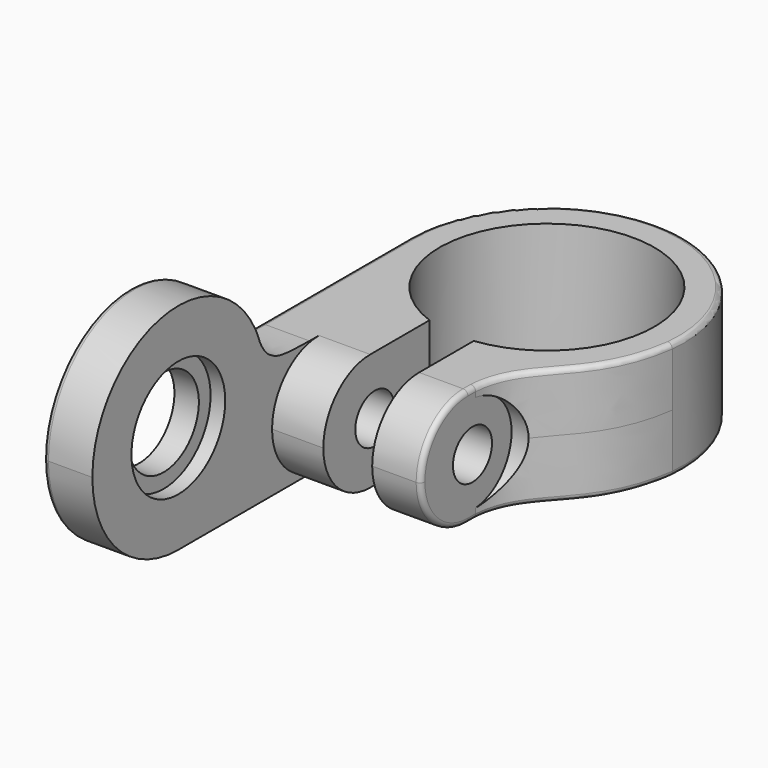
from build123d import *

# Parameters (mm, degrees)
F1_DEPTH     = 6
F3_DEPTH     = 5
F4_R         = 2.5
F5_DEPTH     = 28.0010001
F4_R_2       = 5
F6_DEPTH     = 6
F7_R         = 5
F8_DEPTH     = 7.7510001
F9_R         = 4.5
F10_DEPTH    = 1
F11_DEPTH    = 28.0010001
F12_T1_DEPTH = 5
F12_T3_DEPTH = 5.25
F13_R        = 0.5
F14_R        = 6
F14_R_2      = 4.5
F15_DEPTH    = 1.5


# Not quite as in the source:
# - a fillet or chamfer that OpenCascade refuses, or shapes differently, is made with other operations: its cross-section is extruded or revolved along the edge and cut away or added
# - a feature names something its author has since deleted; it is built from what else it names


with BuildPart() as f1:
    # F0 (on Top) → F1 (new body, symmetric)
    with BuildSketch(Plane.XY):
        with BuildLine():
            ThreePointArc((-3.75, -10.34105894), (1.2840732714, 10.9247954596), (1.25, -10.9287464972))
            Line((1.25, -10.9287464972), (1.25, -23.9287464972))
            Line((1.25, -23.9287464972), (6.25, -23.9287464972))
            Line((6.25, -23.9287464972), (6.25, -16.9424782941))
            add(Edge.make_bspline(
                [(13.9325423216, -1.3726851266), (12.6381972805, -10.4814385995), (6.7273111737, -10.6028057635), (6.25, -16.9424782941)],
                knots=[0, 0, 0, 0, 17.3620251065, 17.3620251065, 17.3620251065, 17.3620251065], degree=3))
            ThreePointArc((13.9325423216, -1.3726851266), (0.6871708294, 13.9831254107), (-14, 0))
            Line((-14, 0), (-14, -23.9287464972))
            Line((-14, -23.9287464972), (-3.75, -23.9287464972))
            Line((-3.75, -23.9287464972), (-3.75, -10.34105894))
        make_face()
    extrude(amount=F1_DEPTH, both=True)

    # F2 (on face) → F3 (join)
    with BuildSketch(Plane(origin=(-14, 0, 0), x_dir=(0, -1, 0), z_dir=(-1, 0, 0))):
        with BuildLine():
            ThreePointArc((35.9287464972, -6), (43.7069210902, -2.7781745931), (46.9287464972, 5))
            ThreePointArc((46.9287464972, 5), (38.4000033429, 15.7188100833), (26.0391302058, 9.8161695992))
            add(Edge.make_bspline(
                [(25.4869740085, 8.4596802299), (25.6594735822, 8.8218641875), (25.8423553432, 9.2659041852), (26.0391302058, 9.8161695992)],
                knots=[0.8880126886, 0.8880126886, 0.8880126886, 0.8880126886, 1, 1, 1, 1], degree=3))
            ThreePointArc((25.4869740085, 8.4596802299), (27.0108856963, -1.4398570431), (35.9287464972, -6))
        make_face()
        with BuildLine():
            add(Edge.make_bspline(
                [(25.4869740085, 8.4596802299), (25.6594735822, 8.8218641875), (25.8423553432, 9.2659041852), (26.0391302058, 9.8161695992)],
                knots=[0.8880126886, 0.8880126886, 0.8880126886, 0.8880126886, 1, 1, 1, 1], degree=3))
            ThreePointArc((26.0391302058, 9.8161695992), (25.7404513363, 9.1471245117), (25.4869740085, 8.4596802299))
        make_face()
        with BuildLine():
            Line((23.9287464972, 6), (23.9287464972, -6))
            Line((23.9287464972, -6), (35.9287464972, -6))
            ThreePointArc((35.9287464972, -6), (27.0108856963, -1.4398570431), (25.4869740085, 8.4596802299))
            add(Edge.make_bspline(
                [(19.1325701837, 6), (22.6899938416, 6), (23.8374523242, 6.4838968901), (24.9481407399, 7.3283338654), (25.4869740085, 8.4596802299)],
                knots=[0, 0, 0, 0, 0.5382002935, 0.8880126886, 0.8880126886, 0.8880126886, 0.8880126886], degree=3))
            Line((19.1325701837, 6), (23.9287464972, 6))
        make_face()
    extrude(amount=-F3_DEPTH)

    # F4 (on face) → F5 (cut, through all)
    with BuildSketch(Plane(origin=(-14, 0, 0), x_dir=(0, -1, 0), z_dir=(-1, 0, 0))):
        with Locations((17.34105894, 0)):
            Circle(F4_R)
    extrude(amount=-F5_DEPTH, mode=Mode.SUBTRACT)

    # F4 (on face) → F6 (cut)
    with BuildSketch(Plane(origin=(-14, 0, 0), x_dir=(0, -1, 0), z_dir=(-1, 0, 0))):
        with Locations((17.34105894, 0)):
            Circle(F4_R_2)
        with Locations((17.34105894, 0)):
            Circle(F4_R, mode=Mode.SUBTRACT)
    extrude(amount=-F6_DEPTH, mode=Mode.SUBTRACT)

    # F7 (on face) → F8 (cut, through all)
    with BuildSketch(Plane.YZ.offset(6.25)):
        with Locations((-17.34105894, 0)):
            Circle(F7_R)
    extrude(amount=F8_DEPTH, mode=Mode.SUBTRACT)

    # F9 (on face) → F10 (cut)
    with BuildSketch(Plane(origin=(-14, 0, 0), x_dir=(0, -1, 0), z_dir=(-1, 0, 0))):
        with BuildLine():
            ThreePointArc((34.4731002269, 12.6120689655), (28.5731123295, 2.5592734708), (39.3124481602, -1.9723068676))
            ThreePointArc((39.3124481602, -1.9723068676), (41.159616015, -2.0143070996), (41.6462424386, -0.231896421))
            ThreePointArc((41.6462424386, -0.231896421), (41.7469365287, -0.1196840486), (41.8454286992, -0.0055341094))
            ThreePointArc((41.8454286992, -0.0055341094), (43.5514595083, 0.7038684435), (43.2748339282, 2.5306884652))
            ThreePointArc((43.2748339282, 2.5306884652), (43.3214793257, 2.6740590451), (43.3653269111, 2.8183098875))
            ThreePointArc((43.3653269111, 2.8183098875), (44.6381060055, 4.1576479629), (43.6455935628, 5.7160805584))
            ThreePointArc((43.6455935628, 5.7160805584), (43.6302034221, 5.8660607565), (43.6118986313, 6.0157131902))
            ThreePointArc((43.6118986313, 6.0157131902), (44.2334947511, 7.7556589846), (42.6950381231, 8.7788619494))
            ThreePointArc((42.6950381231, 8.7788619494), (42.6202476169, 8.9097714466), (42.5429246828, 9.0392012737))
            ThreePointArc((42.5429246828, 9.0392012737), (42.4069051987, 10.8818330338), (40.58592621, 11.1946087142))
            ThreePointArc((40.58592621, 11.1946087142), (40.4645413227, 11.2840325668), (40.341439844, 11.3710781997))
            ThreePointArc((40.341439844, 11.3710781997), (39.4710946558, 13.0008917955), (37.6793899466, 12.5496852592))
            ThreePointArc((37.6793899466, 12.5496852592), (37.5321947731, 12.5823118919), (37.3843927675, 12.6120689655))
            ThreePointArc((37.3843927675, 12.6120689655), (35.9287464972, 13.75), (34.4731002269, 12.6120689655))
        make_face()
        with Locations((35.9287464972, 5)):
            Circle(F9_R, mode=Mode.SUBTRACT)
    extrude(amount=-F10_DEPTH, mode=Mode.SUBTRACT)

    # F11 (cut, through all): a face of the model
    f11_faces = [f1.faces().sort_by_distance(p)[0] for p in [
        (-14, -35.9287464972, 5),
    ]]
    extrude(f11_faces, amount=-F11_DEPTH, mode=Mode.SUBTRACT)

    # F12: fillet of radius 6 on 4 edges, made by hand

    # F12_s2 → F12_t1 (cut)
    with BuildSketch(Plane.YZ.offset(1.25)):
        with BuildLine():
            ThreePointArc((-17.9287464972, -6), (-22.1713871843, -4.2426406871), (-23.9287464972, 0))
            Line((-23.9287464972, 0), (-24.0487464972, 0))
            Line((-24.0487464972, 0), (-24.0487464972, -6.12))
            Line((-24.0487464972, -6.12), (-17.9287464972, -6.12))
            Line((-17.9287464972, -6.12), (-17.9287464972, -6))
        make_face()
        with BuildLine():
            ThreePointArc((-17.9287464972, 6), (-22.1713871843, 4.2426406871), (-23.9287464972, 0))
            Line((-23.9287464972, 0), (-24.0487464972, 0))
            Line((-24.0487464972, 0), (-24.0487464972, 6.12))
            Line((-24.0487464972, 6.12), (-17.9287464972, 6.12))
            Line((-17.9287464972, 6.12), (-17.9287464972, 6))
        make_face()
    extrude(amount=F12_T1_DEPTH, mode=Mode.SUBTRACT)

    # F12_s4 → F12_t3 (cut)
    with BuildSketch(Plane.YZ.offset(-9)):
        with BuildLine():
            ThreePointArc((-17.9287464972, -6), (-22.1713871843, -4.2426406871), (-23.9287464972, 0))
            Line((-23.9287464972, 0), (-24.0487464972, 0))
            Line((-24.0487464972, 0), (-24.0487464972, -6.12))
            Line((-24.0487464972, -6.12), (-17.9287464972, -6.12))
            Line((-17.9287464972, -6.12), (-17.9287464972, -6))
        make_face()
        with BuildLine():
            ThreePointArc((-17.9287464972, 6), (-22.1713871843, 4.2426406871), (-23.9287464972, 0))
            Line((-23.9287464972, 0), (-24.0487464972, 0))
            Line((-24.0487464972, 0), (-24.0487464972, 6.12))
            Line((-24.0487464972, 6.12), (-17.9287464972, 6.12))
            Line((-17.9287464972, 6.12), (-17.9287464972, 6))
        make_face()
    extrude(amount=F12_T3_DEPTH, mode=Mode.SUBTRACT)

    # F13
    f13_edges = [f1.edges().sort_by_distance(p)[0] for p in [
        (6.25, -22.171387, 4.242641),
        (6.25, -17.435612, -6),
        (10.470288, -9.384464, -6),
        (6.25, -17.435612, 6),
        (10.470288, -9.384464, 6),
        (0.687171, 13.983125, -6),
        (0.687171, 13.983125, 6),
        (-14, -17.964373, -6),
        (-14, -44.846607, 11.439857),
        (-14, -22.786929, 6.220362),
        (-14, -9.566285, 6),
    ]]
    fillet(f13_edges, radius=F13_R)

    # F14 (on face) → F15 (cut)
    with BuildSketch(Plane.YZ.offset(-9)):
        with Locations((-35.9287464972, 5)):
            Circle(F14_R)
        with Locations((-35.9287464972, 5)):
            Circle(F14_R_2, mode=Mode.SUBTRACT)
    extrude(amount=-F15_DEPTH, mode=Mode.SUBTRACT)


solid = f1.part
